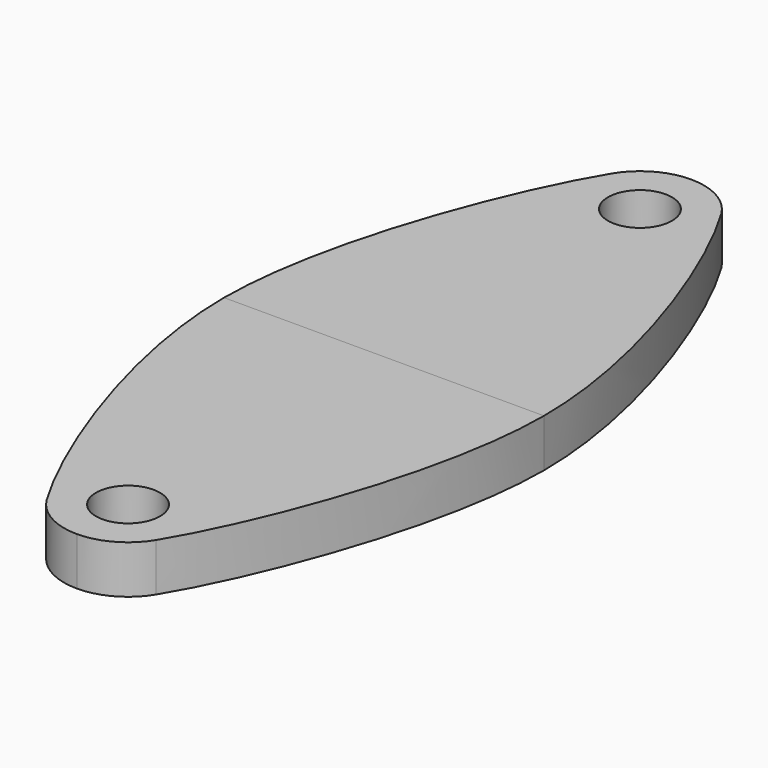
from build123d import *

# Parameters (mm, degrees)
F0_R     = 12.7
F1_DEPTH = 19.05


# Not quite as in the source:
# - a feature names something its author has since deleted; it is built from what else it names


with BuildPart() as f1:
    # F0 (on Top) → F1 (new body)
    with BuildSketch(Plane.XY):
        with BuildLine():
            Line((-63.5, 0), (0, 0))
            Line((0, 0), (63.5, 0))
            add(Edge.make_bspline(
                [(21.6959799399, 140.2077422162), (38.9229681719, 111.9094619356), (63.5, 48.6426617372), (63.5, 0)],
                knots=[0, 0, 0, 0, 146.3071668462, 146.3071668462, 146.3071668462, 146.3071668462], degree=3))
            ThreePointArc((21.6959799399, 140.2077422162), (12.4435394424, 149.1431327085), (0, 152.4))
            ThreePointArc((0, 152.4), (-12.4435394424, 149.1431327085), (-21.6959799399, 140.2077422162))
            add(Edge.make_bspline(
                [(-21.6959799399, 140.2077422162), (-38.9229681719, 111.9094619356), (-63.5, 48.6426617372), (-63.5, 0)],
                knots=[0, 0, 0, 0, 146.3071668462, 146.3071668462, 146.3071668462, 146.3071668462], degree=3))
        make_face()
        with Locations((0, 127)):
            Circle(F0_R, mode=Mode.SUBTRACT)
    extrude(amount=F1_DEPTH)


with BuildPart() as f2_1:
    # F2: instance of F1
    add(f1.part.mirror(Plane.XZ))


solid = Compound([f1.part, f2_1.part])
